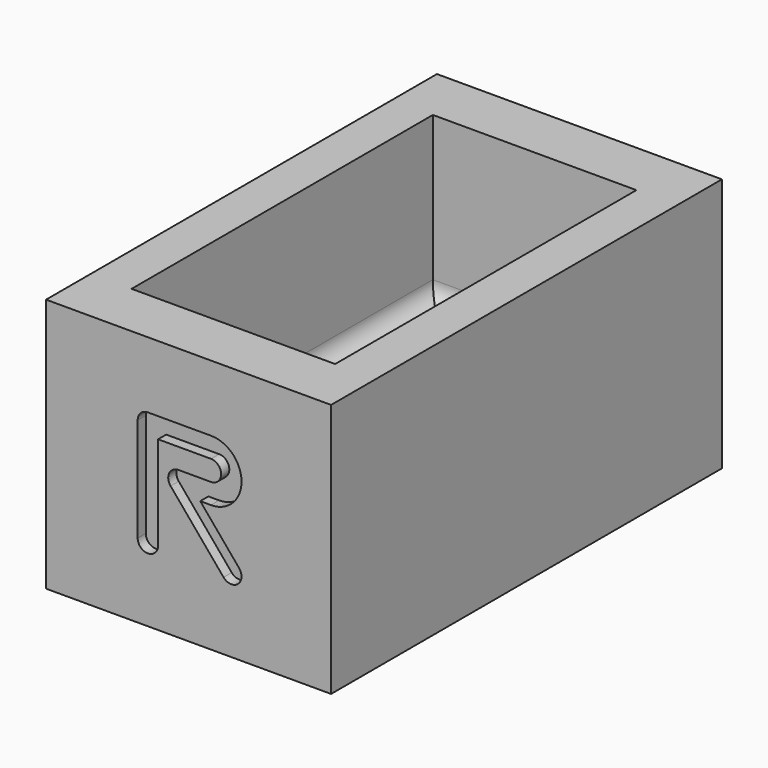
from build123d import *

# Parameters (mm, degrees)
F0_W      = 28
F0_H      = 48
F1_DEPTH  = 25
F2_W      = 20
F2_H      = 37
F3_DEPTH  = 16
F4_R      = 3
F4_R_2    = 1.575
F5_DEPTH  = 2
F6_R      = 5
F6_R_2    = 3
F7_DEPTH  = 4
F8_R      = 4.25
F9_DEPTH  = 3
F10_DEPTH = 9.001
F14_DEPTH = 1
F17_DEPTH = 1
F18_R     = 1.74999


# Not quite as in the source:
# - a fillet or chamfer is up to 0.001 mm smaller than in the source, because OpenCascade refuses the exact size


with BuildPart() as f1:
    # F0 (on Top) → F1 (new body)
    with BuildSketch(Plane.XY):
        with Locations((-14, 24)):
            Rectangle(F0_W, F0_H)
    extrude(amount=F1_DEPTH)

    # F2 (on face) → F3 (cut)
    with BuildSketch(Plane.XY.offset(25)):
        with Locations((-14, 24)):
            Rectangle(F2_W, F2_H)
    extrude(amount=-F3_DEPTH, mode=Mode.SUBTRACT)

    # F4 (on face) → F5 (join)
    with BuildSketch(Plane.XY.offset(9)):
        with Locations((-11, 24)):
            Circle(F4_R)
        with Locations((-11, 24)):
            Circle(F4_R_2, mode=Mode.SUBTRACT)
    extrude(amount=F5_DEPTH)

    # F6 (on face) → F7 (cut)
    with BuildSketch(Plane.XY.offset(9)):
        with Locations((-11, 24)):
            Circle(F6_R)
        with Locations((-11, 24)):
            Circle(F6_R_2, mode=Mode.SUBTRACT)
    extrude(amount=-F7_DEPTH, mode=Mode.SUBTRACT)

    # F8 (on face) → F9 (cut)
    with BuildSketch(Plane(origin=(0, 5.5, 0), x_dir=(-1, 0, 0), z_dir=(0, 1, 0))):
        with Locations((18, 15)):
            Circle(F8_R)
    extrude(amount=-F9_DEPTH, mode=Mode.SUBTRACT)

    # F10 (cut, through all): a face of the model
    f10_faces = [f1.faces().sort_by_distance(p)[0] for p in [
        (-11, 24, 9),
    ]]
    extrude(f10_faces, amount=-F10_DEPTH, mode=Mode.SUBTRACT)

    # F13 (on face) → F14 (cut)
    with BuildSketch(Plane.XZ):
        with BuildLine():
            ThreePointArc((-19, 7.3008629454), (-18, 6.3008629454), (-17, 7.3008629454))
            Line((-17, 7.3008629454), (-17, 16.5))
            Line((-17, 16.5), (-17, 18.5))
            Line((-17, 18.5), (-18, 18.5))
            ThreePointArc((-18, 18.5), (-18.7071067812, 18.2071067812), (-19, 17.5))
            Line((-19, 17.5), (-19, 7.3008629454))
        make_face()
        with BuildLine():
            Line((-17, 18.5), (-17, 16.5))
            Line((-17, 16.5), (-11.7983063839, 16.5))
            ThreePointArc((-11.7983063839, 16.5), (-10.7983063839, 15.5), (-11.7983063839, 14.5))
            Line((-11.7983063839, 14.5), (-15, 14.5))
            ThreePointArc((-15, 14.5), (-14.5773817383, 14.406307787), (-14.2339555569, 14.1427876097))
            Line((-14.2339555569, 14.1427876097), (-12.8554930795, 12.5))
            Line((-12.8554930795, 12.5), (-11.7983063839, 12.5))
            ThreePointArc((-11.7983063839, 12.5), (-8.7983063839, 15.5), (-11.7983063839, 18.5))
            Line((-11.7983063839, 18.5), (-17, 18.5))
        make_face()
        with BuildLine():
            ThreePointArc((-14.2339555569, 14.1427876097), (-14.5773817383, 14.406307787), (-15, 14.5))
            ThreePointArc((-15, 14.5), (-15.906307787, 13.9226182617), (-15.7660444431, 12.8572123903))
            ThreePointArc((-15.7660444431, 12.8572123903), (-15.4226182617, 12.593692213), (-15, 12.5))
            ThreePointArc((-15, 12.5), (-14.2928932188, 12.7928932188), (-14, 13.5))
            ThreePointArc((-14, 13.5), (-14.0603073792, 13.8420201433), (-14.2339555569, 14.1427876097))
        make_face()
        with BuildLine():
            Line((-9.0322619408, 7.9436505551), (-12.8554930795, 12.5))
            Line((-12.8554930795, 12.5), (-15, 12.5))
            ThreePointArc((-15, 12.5), (-15.4226182617, 12.593692213), (-15.7660444431, 12.8572123903))
            Line((-15.7660444431, 12.8572123903), (-10.564350827, 6.6580753357))
            ThreePointArc((-10.564350827, 6.6580753357), (-9.1555187742, 6.5348185023), (-9.0322619408, 7.9436505551))
        make_face()
        with BuildLine():
            Line((-15, 12.5), (-12.8554930795, 12.5))
            Line((-12.8554930795, 12.5), (-14.2339555569, 14.1427876097))
            ThreePointArc((-14.2339555569, 14.1427876097), (-14.0603073792, 13.8420201433), (-14, 13.5))
            ThreePointArc((-14, 13.5), (-14.2928932188, 12.7928932188), (-15, 12.5))
        make_face()
    extrude(amount=-F14_DEPTH, mode=Mode.SUBTRACT)

    # F16 (on face) → F17 (cut)
    with BuildSketch(Plane(origin=(0, 5.5, 0), x_dir=(-1, 0, 0), z_dir=(0, 1, 0))):
        Polygon((9, 14.0925227119), (13.25, 16.5462613559), (13.25, 21.4537386441), (9, 23.9074772881), (4.75, 21.4537386441), (4.75, 16.5462613559), align=None)
        Polygon((9, 14.9585481157), (5.5, 16.9792740578), (5.5, 21.0207259422), (9, 23.0414518843), (12.5, 21.0207259422), (12.5, 16.9792740578), align=None, mode=Mode.SUBTRACT)
        with BuildLine():
            Line((7.5029805213, 17.2914120527), (6.6159696882, 17.7531606659))
            ThreePointArc((6.6159696882, 17.7531606659), (6.8286007981, 17.0787809427), (7.5029805213, 17.2914120527))
        make_face()
        with BuildLine():
            ThreePointArc((8.5564945834, 21.0191256934), (8.5, 21.25), (8.5564945834, 21.4808743066))
            Line((8.5564945834, 21.4808743066), (6.6159696882, 17.7531606659))
            Line((6.6159696882, 17.7531606659), (7.5029805213, 17.2914120527))
            Line((7.5029805213, 17.2914120527), (9, 20.1671597149))
            Line((9, 20.1671597149), (8.5564945834, 21.0191256934))
        make_face()
        with BuildLine():
            Line((9, 20.1671597149), (9.4435054166, 21.0191256934))
            ThreePointArc((9.4435054166, 21.0191256934), (9, 20.75), (8.5564945834, 21.0191256934))
            Line((8.5564945834, 21.0191256934), (9, 20.1671597149))
        make_face()
        with BuildLine():
            ThreePointArc((9.4435054166, 21.0191256934), (9.4856710349, 21.1311570538), (9.5, 21.25))
            ThreePointArc((9.5, 21.25), (9.4856710349, 21.3688429462), (9.4435054166, 21.4808743066))
            ThreePointArc((9.4435054166, 21.4808743066), (9, 21.75), (8.5564945834, 21.4808743066))
            ThreePointArc((8.5564945834, 21.4808743066), (8.5, 21.25), (8.5564945834, 21.0191256934))
            ThreePointArc((8.5564945834, 21.0191256934), (9, 20.75), (9.4435054166, 21.0191256934))
        make_face()
        with BuildLine():
            ThreePointArc((9.4435054166, 21.4808743066), (9.4856710349, 21.3688429462), (9.5, 21.25))
            ThreePointArc((9.5, 21.25), (9.4856710349, 21.1311570538), (9.4435054166, 21.0191256934))
            Line((9.4435054166, 21.0191256934), (9, 20.1671597149))
            Line((9, 20.1671597149), (10.4970194787, 17.2914120527))
            Line((10.4970194787, 17.2914120527), (11.3840303118, 17.7531606659))
            Line((11.3840303118, 17.7531606659), (9.4435054166, 21.4808743066))
        make_face()
        with BuildLine():
            ThreePointArc((10.4970194787, 17.2914120527), (11.1713992019, 17.0787809427), (11.3840303118, 17.7531606659))
            Line((11.3840303118, 17.7531606659), (10.4970194787, 17.2914120527))
        make_face()
    extrude(amount=-F17_DEPTH, mode=Mode.SUBTRACT)

    # F18 (radius 1.75 in the source; OpenCascade refuses exactly that, so slightly less here)
    f18_edges = [f1.edges().sort_by_distance(p)[0] for p in [
        (-24, 24, 9),
        (-14, 42.5, 9),
        (-4, 24, 9),
        (-14, 5.5, 9),
    ]]
    fillet(f18_edges, radius=F18_R)


solid = f1.part
